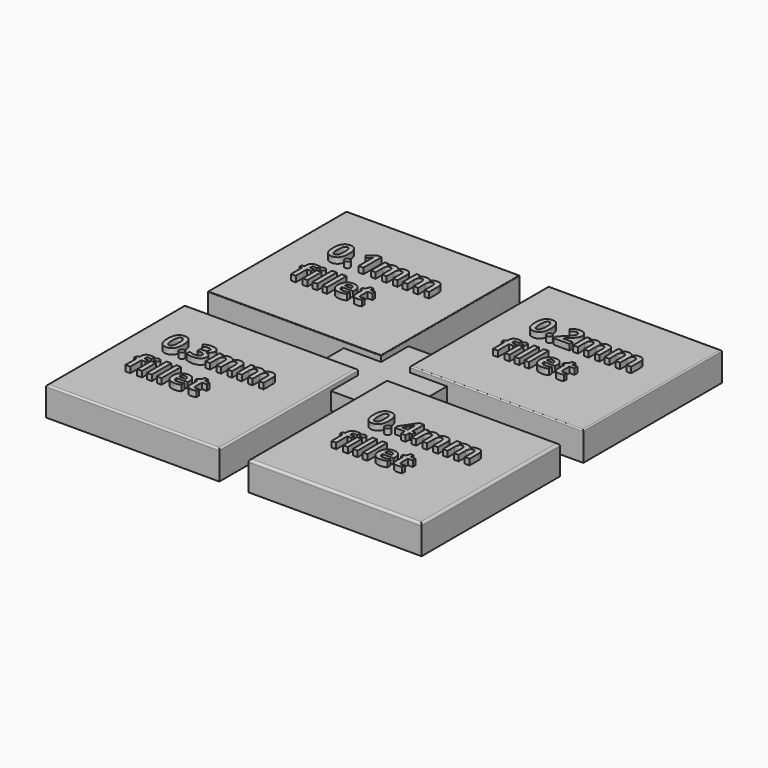
from build123d import *

# Parameters (mm, degrees)
F0_W         = 30
F0_H         = 30
F1_DEPTH     = 5
F2_R         = 0.1
F3_R         = 0.2
F4_R         = 0.3
F5_R         = 0.4
F8_W         = 17.8691577166
F8_H         = 16.7916202918
F9_DEPTH     = 3
F6_TEXT_SIZE = 5.5555555556
F10_DEPTH    = 1


# Not quite as in the source:
# - Text() gives the source's letters only with a copy of the font that has no kerning and outlines rounded to 1/6400 em; it was checked with that copy


with BuildPart() as f1:
    # F0 (on Top) → F1 (new body)
    with BuildSketch(Plane.XY):
        with Locations((-3.6121505499, -4.470018906)):
            Rectangle(F0_W, F0_H)
    extrude(amount=F1_DEPTH)

    # F2
    f2_edges = [f1.edges().sort_by_distance(p)[0] for p in [
        (-3.612151, 10.529981, 5),
        (-18.612151, -4.470019, 5),
        (-3.612151, -19.470019, 5),
        (11.387849, -4.470019, 5),
    ]]
    fillet(f2_edges, radius=F2_R)



with BuildPart() as f1b:
    # F0 (on Top) → F1, piece 2 (new body)
    with BuildSketch(Plane.XY):
        with Locations((31.3878494501, -4.470018906)):
            Rectangle(F0_W, F0_H)
    extrude(amount=F1_DEPTH)

    # F3
    f3_edges = [f1b.edges().sort_by_distance(p)[0] for p in [
        (31.387849, 10.529981, 5),
        (16.387849, -4.470019, 5),
        (31.387849, -19.470019, 5),
        (46.387849, -4.470019, 5),
    ]]
    fillet(f3_edges, radius=F3_R)


with BuildPart() as f1c:
    # F0 (on Top) → F1, piece 3 (new body)
    with BuildSketch(Plane.XY):
        with Locations((31.3878494501, -39.470018906)):
            Rectangle(F0_W, F0_H)
    extrude(amount=F1_DEPTH)

    # F5
    f5_edges = [f1c.edges().sort_by_distance(p)[0] for p in [
        (31.387849, -24.470019, 5),
        (16.387849, -39.470019, 5),
        (31.387849, -54.470019, 5),
        (46.387849, -39.470019, 5),
    ]]
    fillet(f5_edges, radius=F5_R)


with BuildPart() as f1d:
    # F0 (on Top) → F1, piece 4 (new body)
    with BuildSketch(Plane.XY):
        with Locations((-3.6121505499, -39.470018906)):
            Rectangle(F0_W, F0_H)
    extrude(amount=F1_DEPTH)

    # F4
    f4_edges = [f1d.edges().sort_by_distance(p)[0] for p in [
        (11.387849, -39.470019, 5),
        (-3.612151, -24.470019, 5),
        (-18.612151, -39.470019, 5),
        (-3.612151, -54.470019, 5),
    ]]
    fillet(f4_edges, radius=F4_R)


with BuildPart() as f1_1:
    add(f1.part)

    add(f1b.part)  # F9 merges F1b

    add(f1c.part)  # F9 merges F1c

    add(f1d.part)  # F9 merges F1d
    # F8 (on offset) → F9 (join)
    with BuildSketch(Plane.XY.offset(1)):
        with Locations((13.8479294255, -21.9499128871)):
            Rectangle(F8_W, F8_H)
    extrude(amount=F9_DEPTH)

    # F6 (on face) → F10 (join)
    with BuildSketch(Plane.XY.offset(5)):
        with Locations((-12.3752590803, -2.4127906217)):
            Text('0.1mm', F6_TEXT_SIZE, font='Open Sans', font_style=FontStyle.BOLD, text_align=(TextAlign.LEFT, TextAlign.BOTTOM))
        with Locations((-12.3752590803, -9.9683461773)):
            Text('fillet', F6_TEXT_SIZE, font='Open Sans', font_style=FontStyle.BOLD, text_align=(TextAlign.LEFT, TextAlign.BOTTOM))
        with Locations((22.627633065, -2.4480964486)):
            Text('0.2mm', F6_TEXT_SIZE, font='Open Sans', font_style=FontStyle.BOLD, text_align=(TextAlign.LEFT, TextAlign.BOTTOM))
        with Locations((22.627633065, -10.0036520041)):
            Text('fillet', F6_TEXT_SIZE, font='Open Sans', font_style=FontStyle.BOLD, text_align=(TextAlign.LEFT, TextAlign.BOTTOM))
        with Locations((-13.2307757158, -37.1571474671)):
            Text('0.3mm', F6_TEXT_SIZE, font='Open Sans', font_style=FontStyle.BOLD, text_align=(TextAlign.LEFT, TextAlign.BOTTOM))
        with Locations((-13.2307757158, -44.7127030227)):
            Text('fillet', F6_TEXT_SIZE, font='Open Sans', font_style=FontStyle.BOLD, text_align=(TextAlign.LEFT, TextAlign.BOTTOM))
        with Locations((22.4177446216, -37.1571511924)):
            Text('0.4mm', F6_TEXT_SIZE, font='Open Sans', font_style=FontStyle.BOLD, text_align=(TextAlign.LEFT, TextAlign.BOTTOM))
        with Locations((22.4177446216, -44.712706748)):
            Text('fillet', F6_TEXT_SIZE, font='Open Sans', font_style=FontStyle.BOLD, text_align=(TextAlign.LEFT, TextAlign.BOTTOM))
    extrude(amount=F10_DEPTH)


solid = f1_1.part
